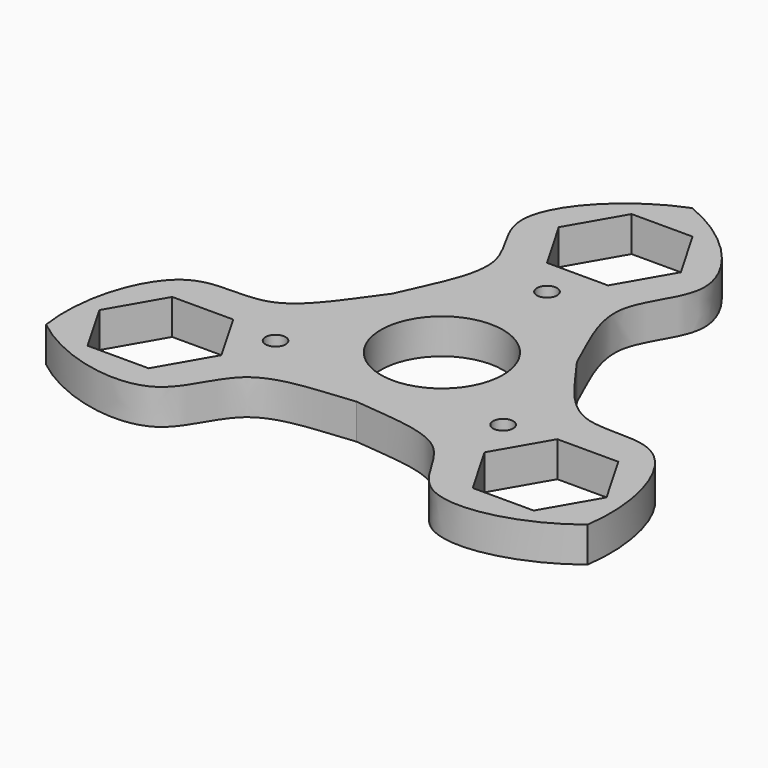
from build123d import *

# Parameters (mm, degrees)
F0_R     = 11
F0_R_2   = 1.8083680483
F1_DEPTH = 6.35
F2_COUNT = 3


# Not quite as in the source:
# - a feature names something its author has since deleted; it is built from what else it names


with BuildPart() as f1:
    # F0 (on Top) → F1 (new body)
    with BuildSketch(Plane.XY):
        with BuildLine():
            ThreePointArc((-16.7417324202, 9.3803920133), (-4.8473828231, -18.5682588984), (19.1905538938, 0))
            ThreePointArc((19.1905538938, 0), (18.5682588984, 4.8473828231), (16.7417324202, 9.3803920133))
            ThreePointArc((16.7417324202, 9.3803920133), (0, 19.1905538938), (-16.7417324202, 9.3803920133))
        make_face()
        Circle(F0_R, mode=Mode.SUBTRACT)
        with BuildLine():
            ThreePointArc((-16.7417324202, 9.3803920133), (0, 19.1905538938), (16.7417324202, 9.3803920133))
            add(Edge.make_bspline(
                [(0, 56.3421584666), (8.906448223, 52.8720755357), (22.0493176942, 38.8214841524), (7.5183827246, 26.377110806), (14.5397577828, 14.7355665073), (16.7417324202, 9.3803920133)],
                knots=[0, 0, 0, 0, 0.3847676827, 0.6735899971, 1, 1, 1, 1], degree=3))
            add(Edge.make_bspline(
                [(0, 56.3421584666), (-8.906448223, 52.8720755357), (-22.0493176942, 38.8214841524), (-7.5183827246, 26.377110806), (-14.5397577828, 14.7355665073), (-16.7417324202, 9.3803920133)],
                knots=[0, 0, 0, 0, 0.3847676827, 0.6735899971, 1, 1, 1, 1], degree=3))
        make_face()
        with Locations((0, 23.6759167165)):
            Circle(F0_R_2, mode=Mode.SUBTRACT)
        Polygon((10.9985226281, 40.0706864893), (5.499261314, 30.5456864893), (-5.499261314, 30.5456864893), (-10.9985226281, 40.0706864893), (-5.499261314, 49.5956864893), (5.499261314, 49.5956864893), align=None, mode=Mode.SUBTRACT)
    extrude(amount=F1_DEPTH)

    # F2: F1 ×3 about axis
    f2_axis = Axis((0, 0, 0), (0, 0, -1))


with BuildPart() as f1_1:
    add(f1.part)
    for i in range(1, F2_COUNT):
        add(f1.part.rotate(f2_axis, i * 360 / F2_COUNT))


solid = f1_1.part
